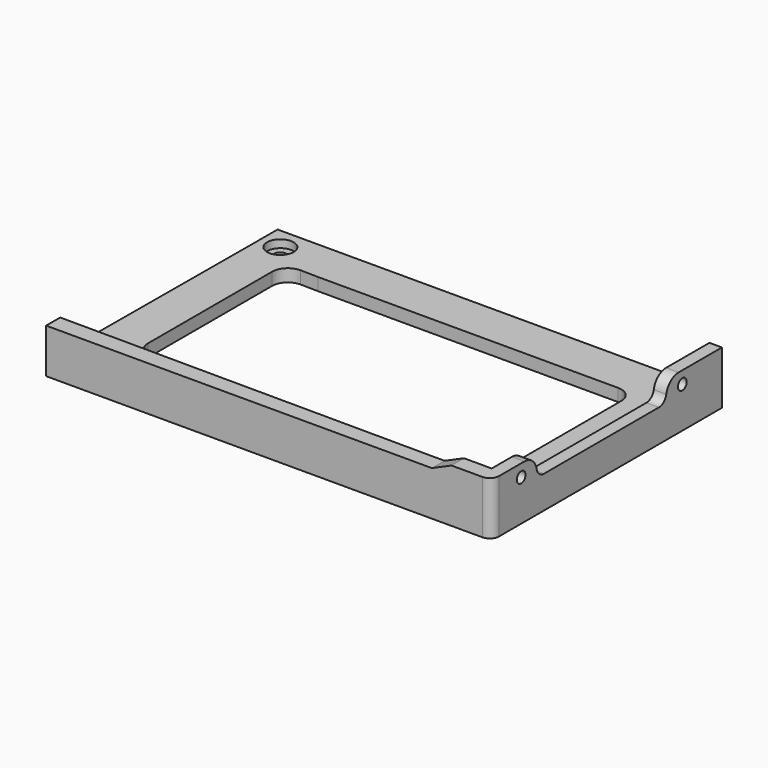
from build123d import *

# Parameters (mm, degrees)
F1_DEPTH  = 17
F3_DEPTH  = 13
F5_R      = 1.75
F6_DEPTH  = 7
F8_DEPTH  = 25
F9_R      = 3
F10_R     = 5
F11_R     = 2
F12_DEPTH = 25
F13_R     = 4.25
F14_DEPTH = 2.5
F16_DEPTH = 25
F17_R     = 5
F18_R     = 3


# Not quite as in the source:
# - ends of sketch curves that miss each other by under 0.0002 mm in the source are joined
# - a feature names something its author has since deleted; it is built from what else it names


with BuildPart() as f1:
    # F0 (on Top) → F1 (new body)
    with BuildSketch(Plane.XY):
        Polygon((67.6393576576, 43.5), (-74.3606423424, 43.5), (-74.7787490059, -48.5), (67.6393576576, -48.5), align=None)
    extrude(amount=F1_DEPTH)

    # F2 (on face) → F3 (cut)
    with BuildSketch(Plane.XY.offset(17)):
        Polygon((63.6393576576, 43.5), (-74.3606423424, 43.5), (-74.7531674957, -42.8710561201), (63.6393576576, -43.5), align=None)
    extrude(amount=-F3_DEPTH, mode=Mode.SUBTRACT)

    # F5 (on face) → F6 (cut)
    with BuildSketch(Plane.YZ.offset(67.6393576576)):
        with Locations((27.6843051805, 13.0568410139)):
            Circle(F5_R)
        with Locations((-36.7146101537, 13.0568410233)):
            Circle(F5_R)
        with BuildLine():
            ThreePointArc((27.6607478596, 17.0567716449), (27.6840839728, 17.0568410078), (27.7074200936, 17.0567742259))
            Line((27.7074200936, 17.0567742259), (47.12958325, 17.057848309))
            Line((47.12958325, 17.057848309), (47.1295543691, 17.7527777587))
            Line((47.1295543691, 17.7527777587), (48.6345604738, 26.1808149253))
            Line((48.6345604738, 26.1808149253), (32.3804893276, 26.9834864621))
            Line((32.3804893276, 26.9834864621), (-57.0169261912, 27.2844880555))
            Line((-57.0169261912, 27.2844880555), (-57.1818195967, 17.0567789567))
            Line((-57.1818195967, 17.0567789567), (-36.7146222837, 17.0568410232))
            Line((-36.7146222837, 17.0568410232), (-30.4415900066, 17.0568410232))
            Line((-30.4415900066, 17.0568410232), (-30.4415900066, 10.3634270296))
            Line((-30.4415900066, 10.3634270296), (21.2007000848, 10.3634270296))
            Line((21.2007000848, 10.3634270296), (21.2007000848, 17.0567742259))
            Line((21.2007000848, 17.0567742259), (27.6607478596, 17.0567716449))
        make_face()
    extrude(amount=-F6_DEPTH, mode=Mode.SUBTRACT)

    # F7 (on face) → F8 (cut)
    with BuildSketch(Plane.XY.offset(4)):
        Polygon((-50.4835, -29.7545), (50.4835, -29.7545), (50.4835, 29.7545), (-50.4835, 29.7545), (-61.1949004233, 29.9527719617), (-61.1949004233, -29.7545), align=None)
    extrude(amount=-F8_DEPTH, mode=Mode.SUBTRACT)

    # F9
    f9_edges = [f1.edges().sort_by_distance(p)[0] for p in [
        (67.639358, -48.5, 8.5),
    ]]
    fillet(f9_edges, radius=F9_R)

    # F10
    f10_edges = [f1.edges().sort_by_distance(p)[0] for p in [
        (50.4835, 29.7545, 2),
        (-61.1949, 29.952772, 2),
        (50.4835, -29.7545, 2),
        (-61.1949, -29.7545, 2),
    ]]
    fillet(f10_edges, radius=F10_R)

    # F11 (on face) → F12 (cut)
    with BuildSketch(Plane.XY.offset(4)):
        with Locations((-67.8764981099, -36.4826410897)):
            Circle(F11_R)
        with Locations((57.0614288288, -36.4826410897)):
            Circle(F11_R)
        with Locations((-67.8764981099, 36.4826410897)):
            Circle(F11_R)
        with Locations((57.0614288288, 36.4826410897)):
            Circle(F11_R)
    extrude(amount=-F12_DEPTH, mode=Mode.SUBTRACT)

    # F13 (on face) → F14 (cut)
    with BuildSketch(Plane.XY.offset(4)):
        with Locations((-67.8764981099, 36.4826410897)):
            Circle(F13_R)
        with Locations((57.0614288288, 36.4826410897)):
            Circle(F13_R)
        with Locations((-67.8764981099, -36.4826410897)):
            Circle(F13_R)
        with Locations((57.0614288288, -36.4826410897)):
            Circle(F13_R)
    extrude(amount=-F14_DEPTH, mode=Mode.SUBTRACT)

    # F15 (on face) → F16 (cut)
    with BuildSketch(Plane.XZ.offset(48.5)):
        Polygon((-78.4085690975, 22.2279634327), (-78.4085690975, 14.2272571102), (48.5201984959, 14.2272571102), (54.7997877002, 17), (47.9935184121, 22.2279634327), align=None)
    extrude(amount=-F16_DEPTH, mode=Mode.SUBTRACT)

    # F17
    f17_edges = [f1.edges().sort_by_distance(p)[0] for p in [
        (65.639358, -30.44159, 17),
        (65.639358, 21.2007, 17),
    ]]
    fillet(f17_edges, radius=F17_R)

    # F18
    f18_edges = [f1.edges().sort_by_distance(p)[0] for p in [
        (65.639358, -30.44159, 10.363427),
        (65.639358, 21.2007, 10.363427),
    ]]
    fillet(f18_edges, radius=F18_R)


solid = f1.part
